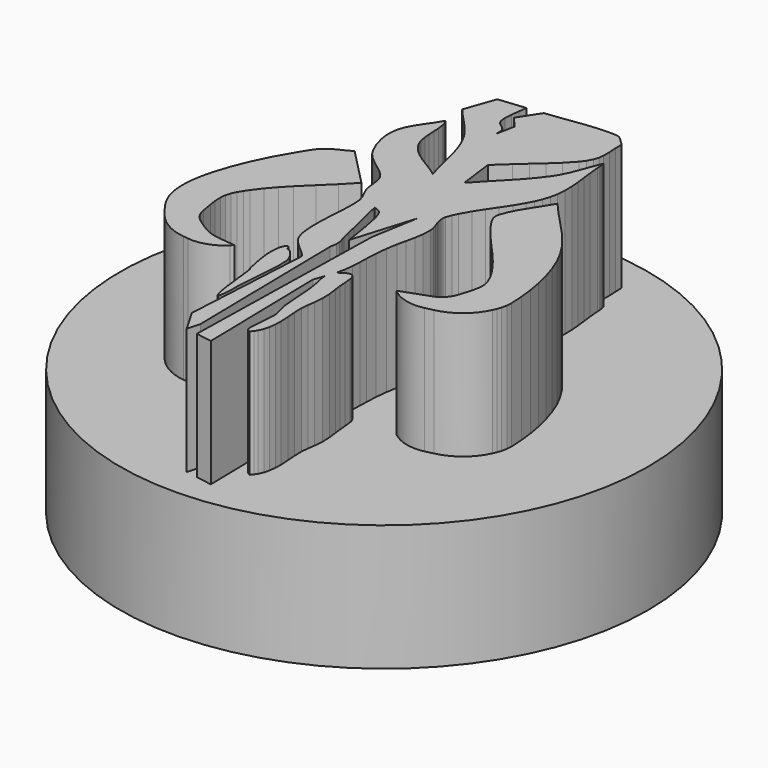
from build123d import *

# Parameters (mm, degrees)
F1_R     = 29.21
F2_DEPTH = 27.94
F0_R     = 29.21
F0_R_2   = 27.94
F0_R_3   = 26.67
F3_DEPTH = 13.97
F4_SCALE = 0.173913


# Not quite as in the source:
# - ends of sketch curves that miss each other by under 0.0002 mm in the source are joined


with BuildPart() as f2:
    # F1 (on face) → F2 (new body)
    with BuildSketch(Plane.XY):
        with Locations((1.0160021484, 2.6811140235)):
            Circle(F1_R)
    extrude(amount=-F2_DEPTH)

    # F0 (on Top) → F3 (cut)
    with BuildSketch(Plane.XY):
        with Locations((1.0160021484, 2.6811140235)):
            Circle(F0_R)
        with Locations((1.0160021484, 2.6811140235)):
            Circle(F0_R_2, mode=Mode.SUBTRACT)
        with Locations((1.0160021484, 2.6811140235)):
            Circle(F0_R_2)
        with Locations((1.0160021484, 2.6811140235)):
            Circle(F0_R_3, mode=Mode.SUBTRACT)
        with Locations((1.0160021484, 2.6811140235)):
            Circle(F0_R_3)
        Polygon((-3.3095653584, -5.6137892885), (-3.1695097584, -5.4395960885), (-3.0529237584, -5.4829538885), (-3.0004219584, -5.5103858885), (-2.9673765584, -5.5440408885), (-2.9427639584, -5.5983460885), (-2.9302163584, -5.6597632885), (-2.9131729584, -5.7589248885), (-2.8898557584, -5.8141190885), (-2.8479203584, -5.8575022885), (-2.7512733584, -5.9104104885), (-2.5523405584, -5.9840196885), (-2.5061633584, -6.0104102885), (-2.4849035584, -6.0263360885), (-2.4798235584, -6.0306286885), (-2.4773343584, -6.0328130885), (-2.4760897584, -6.0339306885), (-2.4754801584, -6.0344894885), (-2.4730163584, -6.0367246885), (-2.4632119584, -6.0456654885), (-2.4242229584, -6.0817588885), (-2.2726103584, -6.2308822885), (-1.9922197584, -6.5571706885), (-1.7587429584, -6.9181808885), (-1.5875723584, -7.3190944885), (-1.4959037584, -7.7449508885), (-1.4564575584, -8.7470316885), (-1.5075115584, -9.7528970885), (-1.5761169584, -10.7580258885), (-1.7809679584, -13.4732858885), (-1.8152833584, -14.2048566885), (-1.8169851584, -14.9385864885), (-1.8529515584, -15.6699794885), (-1.9431723584, -16.2117868885), (-1.9748207584, -16.3335290885), (-2.0227759584, -16.4506738885), (-2.0391081584, -16.4671838885), (-2.0507159584, -16.4732036885), (-2.0637969584, -16.4748800885), (-2.0751253584, -16.4723146885), (-2.0914321584, -16.4626372885), (-2.1228773584, -16.4262898885), (-2.1991789584, -16.2593356885), (-2.3008551584, -15.9096792885), (-2.3766995584, -15.5528854885), (-2.5239687584, -14.6005886885), (-2.6334681584, -13.6423736885), (-2.8588677584, -11.7314300885), (-2.9211739584, -11.2544434885), (-2.9539399584, -11.0161660885), (-2.9707801584, -10.8971162885), (-2.9752505584, -10.8818762885), (-2.9848009584, -10.8691762885), (-3.0330101584, -10.8370960885), (-3.0537111584, -10.8222878885), (-3.0650903584, -10.8089274885), (-3.0688241584, -10.8010026885), (-3.0700179584, -10.7968116885), (-3.0702465584, -10.7957448885), (-3.0703227584, -10.7954908885), (-3.0705259584, -10.7944240885), (-3.0713387584, -10.7901314885), (-3.0746661584, -10.7730372885), (-3.0882551584, -10.7046604885), (-3.1452781584, -10.4317374885), (-3.3700173584, -9.3393850885), (-3.4978301584, -8.5924472885), (-3.5894733584, -7.8403786885), (-3.6277003584, -7.0879798885), (-3.5682897584, -6.3395942885), (-3.5083711584, -6.0704558885), (-3.4161437584, -5.8112742885), align=None, mode=Mode.SUBTRACT)
        with BuildLine():
            Line((-10.3454923584, 11.6649163115), (-9.7154707584, 12.0162745115))
            Line((-9.7154707584, 12.0162745115), (-5.5498707584, 7.7514875115))
            Line((-5.5498707584, 7.7514875115), (-6.9198959584, 6.3156255115))
            Line((-6.9198959584, 6.3156255115), (-8.3367333584, 4.9403933115))
            Line((-8.3367333584, 4.9403933115), (-9.7384831584, 3.5689457115))
            Line((-9.7384831584, 3.5689457115), (-10.6222507584, 2.6428617115))
            Line((-10.6222507584, 2.6428617115), (-11.4586981584, 1.6763409115))
            Line((-11.4586981584, 1.6763409115), (-12.2270481584, 0.6563277115))
            Line((-12.2270481584, 0.6563277115), (-12.5530571584, 0.1778679115))
            Line((-12.5530571584, 0.1778679115), (-12.8566633584, -0.3166700885))
            Line((-12.8566633584, -0.3166700885), (-13.1114253584, -0.8399100885))
            Line((-13.1114253584, -0.8399100885), (-13.2776175584, -1.4147120885))
            Line((-13.2776175584, -1.4147120885), (-13.3395681584, -2.0160824885))
            Line((-13.3395681584, -2.0160824885), (-13.3030175584, -2.8127026885))
            Line((-13.3030175584, -2.8127026885), (-13.1902415584, -3.6027950885))
            Line((-13.1902415584, -3.6027950885), (-12.9876511584, -4.7950710885))
            ThreePointArc((-12.9876511584, -4.7950710885), (-12.6458886406, -5.7381027666), (-11.9657003768, -6.475296573))
            Line((-11.9657003768, -6.475296573), (-11.3262371584, -6.9315412885))
            Line((-11.3262371584, -6.9315412885), (-10.6611889584, -7.3559498885))
            Line((-10.6611889584, -7.3559498885), (-10.1669303584, -7.6130740885))
            Line((-10.1669303584, -7.6130740885), (-9.6479321584, -7.8141404885))
            Line((-9.6479321584, -7.8141404885), (-9.0811311584, -7.9525958885))
            Line((-9.0811311584, -7.9525958885), (-8.5008173584, -8.0379144885))
            Line((-8.5008173584, -8.0379144885), (-7.6721931584, -8.1176704885))
            Line((-7.6721931584, -8.1176704885), (-6.8392255584, -8.2166796885))
            Line((-6.8392255584, -8.2166796885), (-7.1013281584, -8.4787822885))
            ThreePointArc((-7.1013281584, -8.4787822885), (-8.7866271737, -9.5348586077), (-10.7637806827, -9.7502650449))
            Line((-10.7637806827, -9.7502650449), (-11.2680457584, -9.6909210885))
            ThreePointArc((-11.2680457584, -9.6909210885), (-13.3569404423, -9.0212773173), (-15.0397067215, -7.6140816273))
            Line((-15.0397067215, -7.6140816273), (-15.6487329584, -6.8493722885))
            Line((-15.6487329584, -6.8493722885), (-16.2212997584, -6.0557746885))
            Line((-16.2212997584, -6.0557746885), (-16.5837323584, -5.4619734885))
            Line((-16.5837323584, -5.4619734885), (-16.8932567584, -4.8286244885))
            Line((-16.8932567584, -4.8286244885), (-17.1266827584, -4.1564896885))
            Line((-17.1266827584, -4.1564896885), (-17.2765935584, -3.4465596885))
            Line((-17.2765935584, -3.4465596885), (-17.3543429584, -2.7171224885))
            Line((-17.3543429584, -2.7171224885), (-17.3680335584, -1.9835704885))
            Line((-17.3680335584, -1.9835704885), (-17.2836039584, -0.8674944885))
            Line((-17.2836039584, -0.8674944885), (-17.0950851584, 0.2349671115))
            Line((-17.0950851584, 0.2349671115), (-16.8279279584, 1.3131463115))
            Line((-16.8279279584, 1.3131463115), (-16.2564787584, 3.0786749115))
            Line((-16.2564787584, 3.0786749115), (-15.5659289584, 4.7901777115))
            Line((-15.5659289584, 4.7901777115), (-14.6148767584, 6.7561885115))
            Line((-14.6148767584, 6.7561885115), (-13.5328367584, 8.6467105115))
            Line((-13.5328367584, 8.6467105115), (-13.2243791584, 9.1616955115))
            Line((-13.2243791584, 9.1616955115), (-12.9099017584, 9.6756391115))
            Line((-12.9099017584, 9.6756391115), (-12.5667223584, 10.1631921115))
            Line((-12.5667223584, 10.1631921115), (-12.1721841584, 10.5990307115))
            Line((-12.1721841584, 10.5990307115), (-11.8060939584, 10.8919181115))
            Line((-11.8060939584, 10.8919181115), (-11.4065011584, 11.1371297115))
            Line((-11.4065011584, 11.1371297115), (-10.9902459584, 11.3523693115))
            Line((-10.9902459584, 11.3523693115), (-10.3454923584, 11.6649163115))
        make_face(mode=Mode.SUBTRACT)
        Polygon((8.0661040416, 22.4261343115), (8.5338704416, 23.6204931115), (8.5923920416, 23.3269199115), (8.6183762416, 23.1795237115), (8.6328542416, 23.0303495115), (8.6330320416, 23.0256759115), (8.6337686416, 23.0069815115), (8.6369182416, 22.9321785115), (8.6535298416, 22.6331443115), (8.7672202416, 21.4402841115), (8.8865494416, 20.4831359115), (9.0008240416, 19.5213649115), (9.0800466416, 18.5585525115), (9.0942960416, 17.5982801115), (9.0136510416, 16.6440783115), (8.8528182416, 15.8703435115), (8.6087496416, 15.1157857115), (8.2981838416, 14.3845705115), (7.9378594416, 13.6808635115), (7.3038500416, 12.6231059115), (6.6187358416, 11.5943551115), (5.9217598416, 10.5717511115), (5.2521396416, 9.5324847115), (4.6490674416, 8.4536959115), (4.3606504416, 7.8614949115), (4.1353270416, 7.2449861115), (4.0925788416, 6.9641129115), (4.1026118416, 6.6794043115), (4.1737572416, 6.3142539115), (4.2830534416, 5.9577649115), (4.4482042416, 5.4897191115), (4.5931874416, 5.0155011115), (4.6662124416, 4.5302087115), (4.6287728416, 3.5591413115), (4.4759664416, 2.5943477115), (4.2646130416, 1.6343293115), (4.0514562416, 0.6775875115), (3.8455384416, -0.5475052885), (3.7179542416, -1.7848408885), (3.6589754416, -3.0265960885), (3.6352772416, -3.9616462885), (3.5841724416, -4.8977124885), (3.4727934416, -5.8243806885), (3.2682218416, -6.7312368885), (3.4414752416, -6.6185370885), (3.5283686416, -6.5629110885), (3.5707612416, -6.5335232885), (3.5733774416, -6.5316436885), (3.5746728416, -6.5306784885), (3.5799052416, -6.5268938885), (3.6008348416, -6.5118316885), (3.6855692416, -6.4529798885), (4.0465286416, -6.2508466885), (4.2873714416, -6.1790154885), (4.4545034416, -6.1779740885), (4.5851610416, -6.2217382885), (4.6940762416, -6.3064980885), (4.8063442416, -6.4761446885), (4.8911802416, -6.7184860885), (4.9391100416, -6.9721812885), (5.0166562416, -7.7150550885), (5.0728664416, -8.4605704885), (5.1635952416, -9.2012852885), (5.2942782416, -10.2066934885), (5.3297366416, -11.2217536885), (5.2487614416, -12.2298542885), (5.1341820416, -13.0151714885), (5.0642558416, -13.8045526885), (5.0875984416, -14.8106212885), (5.1678370416, -15.8161056885), (5.2228026416, -16.8224536885), (5.2067498416, -17.5585964885), (5.1168084416, -18.2882368885), (4.9692344416, -18.8575778885), (4.7352242416, -19.3954228885), (4.5239978416, -19.7238702885), (4.2690834416, -20.0192468885), (4.0580856416, -19.8658054885), (3.9541234416, -19.7850080885), (3.8989800416, -19.7162756885), (3.8755612416, -19.6531312885), (3.8732244416, -19.6366466885), (3.8725894416, -19.6283662885), (3.8724116416, -19.6242260885), (3.8723608416, -19.6231846885), (3.8722592416, -19.6190190885), (3.8718274416, -19.6024074885), (3.8704558416, -19.5359102885), (3.8697954416, -19.2698960885), (3.9251420416, -18.2064742885), (4.0465540416, -16.7551944885), (4.0697696416, -16.3887740885), (4.0461222416, -16.0254270885), (3.9571714416, -15.6713764885), (3.8490182416, -15.3222534885), (3.6780762416, -14.5939846885), (3.5841724416, -13.8480882885), (3.5269716416, -13.0982548885), (3.3674088416, -10.8850766885), (3.2837920416, -10.1266326885), (3.1492482416, -9.3764690885), (3.0318748416, -8.8792132885), (2.9315194416, -8.3784522885), (2.8809226416, -7.8725096885), (2.4838190416, -9.0101248885), (2.7813546416, -23.4905886885), (0.9960902416, -23.1930276885), (1.4919998416, 0.4120813115), (2.3846320416, 5.5695005115), (0.3018320416, -1.2739960885), (0.0915962416, 0.0695877115), (-0.1240497584, 1.4122063115), (-0.3820375584, 2.7475605115), (-0.5009857584, 3.3255629115), (-0.6647141584, 3.8912463115), (-0.8834081584, 4.3707475115), (-1.0111701584, 4.5227411115), (-1.2562801584, 4.6632285115), (-1.5219895584, 4.7624409115), (-1.7809679584, 4.8752423115), (-0.8256231584, 0.8472595115), (-0.5964389584, -0.1624666885), (-0.3547833584, -1.1691702885), (-0.2221445584, -1.6122224885), (-0.1035011584, -2.0585512885), (-0.0757135584, -2.5098838885), (-0.1940775584, -3.2576090885), (0.1034580416, -21.6061372885), (-0.2932645584, -22.9946790885), (-1.7809679584, -20.4159694885), (-0.9875227584, -6.1338796885), (-1.4807907584, -5.6341092885), (-2.0100251584, -5.1712450885), (-2.5597827584, -4.6838952885), (-3.0595785584, -4.1487426885), (-3.3074317584, -3.7897898885), (-3.4946043584, -3.3963946885), (-3.6684419584, -2.7556034885), (-3.7596025584, -2.0930952885), (-3.8050431584, -1.4256848885), (-3.8107073584, 0.0444671115), (-3.7281065584, 1.5153049115), (-3.6398415584, 2.9859141115), (-3.6105553584, 3.7217013115), (-3.6112157584, 4.4578695115), (-3.6794909584, 5.1880179115), (-3.7738265584, 5.5503997115), (-3.9207401584, 5.8981511115), (-4.0918345584, 6.2345487115), (-4.2959743584, 6.6588811115), (-4.4605155584, 7.1009173115), (-4.5651635584, 7.5582697115), (-4.6428367584, 8.2881133115), (-4.7504565584, 9.0121149115), (-4.8538599584, 9.3518399115), (-5.0104255584, 9.6688065115), (-5.2961247584, 10.0398243115), (-5.6347829584, 10.3630901115), (-6.1587595584, 10.7813519115), (-6.7016083584, 11.1859485115), (-7.2371673584, 11.5971491115), (-7.7392491584, 12.0351721115), (-8.1817171584, 12.5202613115), (-8.5384093584, 13.0726605115), (-8.9882687584, 14.0837075115), (-9.3054893584, 15.1465451115), (-9.4336069584, 15.9750931115), (-9.4430303584, 16.8133439115), (-9.3338611584, 17.5000329115), (-9.1114079584, 18.1563181115), (-8.6753153584, 18.9827579115), (-8.1585523584, 19.7639603115), (-7.6245427584, 20.5370855115), (-7.1367611584, 21.3393191115), (-6.9672161584, 21.0473969115), (-6.8895937584, 20.8973845115), (-6.8592407584, 20.8183397115), (-6.8472011584, 20.7777251115), (-6.8420957584, 20.7571765115), (-6.8397843584, 20.7468387115), (-6.8392255584, 20.7442479115), (-6.8370411584, 20.7338847115), (-6.8285321584, 20.6923557115), (-6.7977981584, 20.5255285115), (-6.7172547584, 19.8507013115), (-6.6781387584, 19.1706163115), (-6.6455251584, 18.4886771115), (-6.5838539584, 17.8118941115), (-6.4574889584, 17.1472777115), (-6.2646013584, 16.5940657115), (-5.9806547584, 16.0841861115), (-5.4611993584, 15.4630291115), (-4.8518533584, 14.9281305115), (-4.1021977584, 14.4026553115), (-3.3204365584, 13.9190393115), (-2.5366433584, 13.4351693115), (-1.7809679584, 12.9089067115), (-2.2346119584, 14.6381387115), (-2.6529245584, 16.3778355115), (-2.9137317584, 17.3361521115), (-3.2208431584, 18.2799907115), (-3.6013097584, 19.2175301115), (-4.0769247584, 20.1075715115), (-4.5533017584, 20.7934985115), (-5.0823583584, 21.4401063115), (-5.6411837584, 22.0585709115), (-6.5040725584, 22.9759681115), (-7.3351097584, 23.9180287115), (-6.1449419584, 27.2901835115), (-3.1695097584, 27.5877191115), (-3.2667409584, 26.7103777115), (-3.3875941584, 25.8349667115), (-3.4357779584, 24.9566855115), (-3.3797963584, 24.3776417115), (-3.2721765584, 24.0808427115), (-3.1520091584, 23.9295349115), (-3.0097437584, 23.7978613115), (-2.6839125584, 23.5469601115), (-2.3816525584, 23.2716749115), (-2.2410635584, 23.0499329115), (-2.1877997584, 22.7911323115), (-2.1856915584, 22.5112751115), (-2.1776905584, 22.2319513115), (-1.7809679584, 24.2155643115), (-2.8719741584, 25.5049191115), (-1.3842453584, 27.7860931115), (0.5081562416, 28.0123817115), (2.3984242416, 28.2699377115), (3.3428470416, 28.3786751115), (4.2880572416, 28.4573897115), (5.2325054416, 28.4933815115), (5.9890698416, 28.4830945115), (6.1937684416, 28.4589391115), (6.3889166416, 28.3953375115), (6.6050706416, 28.2646799115), (6.7997362416, 28.1014849115), (7.1619402416, 27.7336167115), (7.5420512416, 27.3893705115), (7.5523890416, 26.5162455115), (7.6090818416, 25.6425363115), (7.6128410416, 24.7698177115), (7.5422290416, 24.2320743115), (7.3854094416, 23.7152351115), (7.0637184416, 23.1157189115), (6.6520098416, 22.5731495115), (5.6734494416, 21.5312669115), (4.6261312416, 20.5515127115), (3.5477488416, 19.5987079115), (2.4760212416, 18.6376481115), (0.8969286416, 17.1737191115), (1.3928128416, 13.3056293115), (2.7371586416, 14.7357255115), (4.1018752416, 16.1440285115), (4.9437836416, 17.0521039115), (5.7479984416, 17.9923611115), (6.4934884416, 18.9767127115), (6.9340006416, 19.6884715115), (7.3056534416, 20.4422673115), (7.6250330416, 21.2196851115), align=None, mode=Mode.SUBTRACT)
        with BuildLine():
            ThreePointArc((13.3561343411, -7.132521402), (11.3316611954, -7.1213781471), (9.5221088802, -6.2135587222))
            Line((9.5221088802, -6.2135587222), (9.4265026416, -6.1338796885))
            Line((9.4265026416, -6.1338796885), (12.5173270416, -5.0099296885))
            ThreePointArc((12.5173270416, -5.0099296885), (13.4896977223, -4.3734525934), (14.0767872311, -3.3704872396))
            Line((14.0767872311, -3.3704872396), (14.1046746416, -3.2805706885))
            Line((14.1046746416, -3.2805706885), (14.3008134416, -2.6644682885))
            Line((14.3008134416, -2.6644682885), (14.4844808416, -2.0442256885))
            Line((14.4844808416, -2.0442256885), (14.6265176416, -1.4026724885))
            Line((14.6265176416, -1.4026724885), (14.6799846416, -0.7477334885))
            Line((14.6799846416, -0.7477334885), (14.6443738416, -0.3363042885))
            Line((14.6443738416, -0.3363042885), (14.5441200416, 0.0614851115))
            Line((14.5441200416, 0.0614851115), (14.2042172416, 0.8476659115))
            Line((14.2042172416, 0.8476659115), (13.7782338416, 1.5889649115))
            Line((13.7782338416, 1.5889649115), (13.3048032416, 2.2973963115))
            Line((13.3048032416, 2.2973963115), (12.5176064416, 3.3441811115))
            Line((12.5176064416, 3.3441811115), (11.6722436416, 4.3474049115))
            Line((11.6722436416, 4.3474049115), (10.7968326416, 5.3292419115))
            Line((10.7968326416, 5.3292419115), (9.4878436416, 6.8087919115))
            Line((9.4878436416, 6.8087919115), (8.4190370416, 8.1488451115))
            Line((8.4190370416, 8.1488451115), (7.9258706416, 8.8534157115))
            Line((7.9258706416, 8.8534157115), (7.6935114416, 9.2257289115))
            Line((7.6935114416, 9.2257289115), (7.5055514416, 9.6219943115))
            Line((7.5055514416, 9.6219943115), (7.4370730416, 9.8464033115))
            Line((7.4370730416, 9.8464033115), (7.4034180416, 10.0783561115))
            Line((7.4034180416, 10.0783561115), (7.4201312416, 10.3152111115))
            Line((7.4201312416, 10.3152111115), (7.4785512416, 10.5465797115))
            Line((7.4785512416, 10.5465797115), (7.7880756416, 11.3548839115))
            Line((7.7880756416, 11.3548839115), (8.1760606416, 12.1276789115))
            Line((8.1760606416, 12.1276789115), (8.8142864416, 13.1896275115))
            Line((8.8142864416, 13.1896275115), (9.4846940416, 14.2297575115))
            Line((9.4846940416, 14.2297575115), (10.1207608416, 15.2892677115))
            Line((10.1207608416, 15.2892677115), (11.3126304416, 13.9281579115))
            Line((11.3126304416, 13.9281579115), (12.5453432416, 12.6205913115))
            Line((12.5453432416, 12.6205913115), (13.7624604416, 11.3159203115))
            Line((13.7624604416, 11.3159203115), (14.6354330416, 10.2954499115))
            Line((14.6354330416, 10.2954499115), (15.4457184416, 9.2193535115))
            Line((15.4457184416, 9.2193535115), (16.1708122416, 8.0821193115))
            Line((16.1708122416, 8.0821193115), (16.7882354416, 6.8782863115))
            Line((16.7882354416, 6.8782863115), (17.3346656416, 5.5204023115))
            Line((17.3346656416, 5.5204023115), (17.7829756416, 4.1131661115))
            Line((17.7829756416, 4.1131661115), (18.1356546416, 2.6702175115))
            Line((18.1356546416, 2.6702175115), (18.3951410416, 1.2052471115))
            Line((18.3951410416, 1.2052471115), (18.5628318416, -0.2451436885))
            Line((18.5628318416, -0.2451436885), (18.6484298416, -1.7055674885))
            Line((18.6484298416, -1.7055674885), (18.6148510416, -2.3249464885))
            Line((18.6148510416, -2.3249464885), (18.4841680416, -2.9266724885))
            Line((18.4841680416, -2.9266724885), (18.3346636416, -3.3551958885))
            Line((18.3346636416, -3.3551958885), (18.1562032416, -3.7687078885))
            ThreePointArc((18.1562032416, -3.7687078885), (16.5671418558, -5.8024333082), (14.2454107654, -6.9296893542))
            Line((14.2454107654, -6.9296893542), (13.3561343411, -7.132521402))
        make_face(mode=Mode.SUBTRACT)
    extrude(amount=-F3_DEPTH, mode=Mode.SUBTRACT)


with BuildPart() as f2_1:
    # F4: moved
    add(f2.part.scale(F4_SCALE))


solid = f2_1.part
